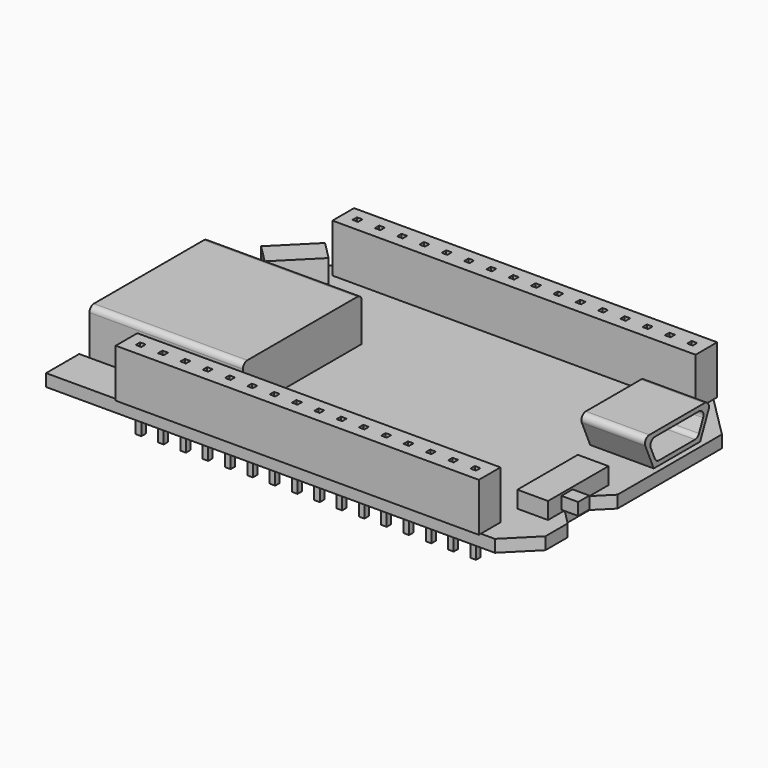
from build123d import *

# Parameters (mm, degrees)
F1_DEPTH  = 1.1
F3_DEPTH  = 1.101
F4_R      = 0.4
F5_DEPTH  = 1.101
F6_W      = 32.55
F6_H      = 2.42
F7_DEPTH  = 4.34
F9_DEPTH  = 2.05
F14_W     = 13.32
F14_H     = 5.65
F15_DEPTH = 9.676
F16_W     = 13.32
F16_H     = 3.93
F17_DEPTH = 4.074
F18_W     = 12.66
F18_H     = 4.99
F18_W_2   = 10.7
F18_H_2   = 2
F19_DEPTH = 8.62
F20_SIZE  = 0.5
F21_R     = 0.5
F11_W     = 2.75
F11_H     = 6.77
F22_DEPTH = 1.5
F26_DEPTH = 5.7
F28_DEPTH = 4
F29_W     = 3.7
F29_H     = 0.8
F30_DEPTH = 2.5
F31_R     = 0.5
F32_W     = 1
F32_H     = 1.45
F33_DEPTH = 0.35
F35_W     = 0.5
F35_H     = 0.5
F36_DEPTH = 3
F37_W     = 0.5
F37_H     = 0.5
F38_DEPTH = 2.7
F39_W     = 1.85
F39_H     = 0.9
F40_DEPTH = 0.7
F41_W     = 1.25
F41_H     = 1.1
F42_DEPTH = 1.5


with BuildPart() as f1:
    # F0 (on Top) → F1 (new body)
    with BuildSketch(Plane.XY):
        Polygon((6.593, 26.37), (0, 19.777), (0, 17.449), (10.426, 17.449), (10.426, 3.714), (0, 3.714), (0, 0), (40.224, 0), (42.743, 2.519), (42.743, 5.019), (41.349, 6.413), (41.349, 9.202), (42.743, 10.596), (42.743, 22.296), (38.669, 26.37), align=None)
    extrude(amount=-F1_DEPTH)

    # F2 (on face) → F3 (cut, through all)
    with BuildSketch(Plane.XY):
        with BuildLine():
            Line((10.426, 16.449), (10.926, 16.449))
            ThreePointArc((10.926, 16.449), (11.426, 16.949), (10.926, 17.449))
            Line((10.926, 17.449), (10.426, 17.449))
            Line((10.426, 17.449), (10.426, 16.449))
        make_face()
        with BuildLine():
            Line((10.426, 3.714), (10.926, 3.714))
            ThreePointArc((10.926, 3.714), (11.426, 4.214), (10.926, 4.714))
            Line((10.926, 4.714), (10.426, 4.714))
            Line((10.426, 4.714), (10.426, 3.714))
        make_face()
    extrude(amount=-F3_DEPTH, mode=Mode.SUBTRACT)

    # F4 (on face) → F5 (cut, through all)
    with BuildSketch(Plane.XY):
        with Locations((7.694, 0.99)):
            Circle(F4_R)
        with Locations((7.694, 25.272)):
            Circle(F4_R)
        with Locations((9.694, 0.99)):
            Circle(F4_R)
        with Locations((9.694, 25.272)):
            Circle(F4_R)
        with Locations((11.694, 0.99)):
            Circle(F4_R)
        with Locations((11.694, 25.272)):
            Circle(F4_R)
        with Locations((13.694, 0.99)):
            Circle(F4_R)
        with Locations((13.694, 25.272)):
            Circle(F4_R)
        with Locations((15.694, 0.99)):
            Circle(F4_R)
        with Locations((15.694, 25.272)):
            Circle(F4_R)
        with Locations((17.694, 0.99)):
            Circle(F4_R)
        with Locations((17.694, 25.272)):
            Circle(F4_R)
        with Locations((19.694, 0.99)):
            Circle(F4_R)
        with Locations((19.694, 25.272)):
            Circle(F4_R)
        with Locations((21.694, 0.99)):
            Circle(F4_R)
        with Locations((21.694, 25.272)):
            Circle(F4_R)
        with Locations((23.694, 0.99)):
            Circle(F4_R)
        with Locations((23.694, 25.272)):
            Circle(F4_R)
        with Locations((25.694, 0.99)):
            Circle(F4_R)
        with Locations((25.694, 25.272)):
            Circle(F4_R)
        with Locations((27.694, 0.99)):
            Circle(F4_R)
        with Locations((27.694, 25.272)):
            Circle(F4_R)
        with Locations((29.694, 0.99)):
            Circle(F4_R)
        with Locations((29.694, 25.272)):
            Circle(F4_R)
        with Locations((31.694, 0.99)):
            Circle(F4_R)
        with Locations((31.694, 25.272)):
            Circle(F4_R)
        with Locations((33.694, 0.99)):
            Circle(F4_R)
        with Locations((33.694, 25.272)):
            Circle(F4_R)
        with Locations((35.694, 0.99)):
            Circle(F4_R)
        with Locations((35.694, 25.272)):
            Circle(F4_R)
        with Locations((37.694, 0.99)):
            Circle(F4_R)
        with Locations((37.694, 25.272)):
            Circle(F4_R)
    extrude(amount=-F5_DEPTH, mode=Mode.SUBTRACT)

    # F25 (on plane+point) → F26 (join, through all)
    with BuildSketch(Plane.YZ.offset(42.243)):
        Polygon((21.734, 2.85), (14.034, 2.85), (15.284, 0), (20.484, 0), align=None)
    extrude(amount=-F26_DEPTH)

    # F27 (on face) → F28 (cut)
    with BuildSketch(Plane.YZ.offset(42.243)):
        Polygon((20.222656384, 0.4), (21.121779191, 2.45), (14.646220809, 2.45), (15.545343616, 0.4), align=None)
    extrude(amount=-F28_DEPTH, mode=Mode.SUBTRACT)

    # F29 (on face) → F30 (join)
    with BuildSketch(Plane.YZ.offset(38.243)):
        with Locations((17.884, 1.8)):
            Rectangle(F29_W, F29_H)
    extrude(amount=F30_DEPTH)

    # F31
    f31_edges = [f1.edges().sort_by_distance(p)[0] for p in [
        (39.393, 14.034, 2.85),
        (39.393, 21.734, 2.85),
        (40.243, 21.121779, 2.45),
        (40.243, 14.646221, 2.45),
        (40.243, 20.222656, 0.4),
        (40.243, 15.545344, 0.4),
    ]]
    fillet(f31_edges, radius=F31_R)


with BuildPart() as f7:
    # F6 (on face) → F7 (new body)
    with BuildSketch(Plane.XY):
        with Locations((22.694, 0.99)):
            Rectangle(F6_W, F6_H)
    extrude(amount=F7_DEPTH)


with BuildPart() as f7b:
    # F6 (on face) → F7, piece 2 (new body)
    with BuildSketch(Plane.XY):
        with Locations((22.694, 25.272)):
            Rectangle(F6_W, F6_H)
    extrude(amount=F7_DEPTH)


with BuildPart() as f9:
    # F8 (on face) → F9 (new body)
    with BuildSketch(Plane.XY):
        Polygon((5.3819805153, 24.5239805153), (2.2, 21.342), (3.8263455967, 19.7156544033), (7.0083261121, 22.8976349186), align=None)
    extrude(amount=F9_DEPTH)

    # F39 (on face) → F40 (join)
    with BuildSketch(Plane(origin=(-9.571, 9.571, 0), x_dir=(-0.7071067812, -0.7071067812, 0), z_dir=(-0.7071067812, 0.7071067812, 0))):
        with Locations((-18.8967078427, 1.025)):
            Rectangle(F39_W, F39_H)
    extrude(amount=F40_DEPTH)


with BuildPart() as f15:
    # F14 (on offset) → F15 (new body, through all)
    with BuildSketch(Plane(origin=(0.75, 0, 0), x_dir=(0, -1, 0), z_dir=(-1, 0, 0))):
        with Locations((-10.5815, 1.105)):
            Rectangle(F14_W, F14_H)
    extrude(amount=-F15_DEPTH)

    # F16 (on face) → F17 (join, through all)
    with BuildSketch(Plane.YZ.offset(10.426)):
        with Locations((10.5815, 1.965)):
            Rectangle(F16_W, F16_H)
    extrude(amount=F17_DEPTH)

    # F18 (on face) → F19 (cut)
    with BuildSketch(Plane(origin=(0.75, 0, 0), x_dir=(0, -1, 0), z_dir=(-1, 0, 0))):
        with Locations((-10.5815, 1.105)):
            Rectangle(F18_W, F18_H)
        with Locations((-10.5815, 2.31)):
            Rectangle(F18_W_2, F18_H_2, mode=Mode.SUBTRACT)
    extrude(amount=-F19_DEPTH, mode=Mode.SUBTRACT)

    # F20
    f20_edges = [f15.edges().sort_by_distance(p)[0] for p in [
        (0.75, 15.9315, 2.31),
        (0.75, 10.5815, 3.31),
        (0.75, 10.5815, 1.31),
        (0.75, 5.2315, 2.31),
    ]]
    chamfer(f20_edges, length=F20_SIZE)

    # F21
    f21_edges = [f15.edges().sort_by_distance(p)[0] for p in [
        (7.625, 17.2415, 3.93),
        (5.06, 16.9115, 3.6),
        (7.625, 3.9215, 3.93),
        (5.06, 4.2515, 3.6),
        (5.06, 4.2515, -1.39),
        (5.06, 16.9115, -1.39),
        (5.588, 17.2415, -1.72),
        (5.588, 3.9215, -1.72),
    ]]
    fillet(f21_edges, radius=F21_R)

    # F32 (on face) → F33 (join)
    with BuildSketch(Plane(origin=(0, 0, -1.72), x_dir=(1, 0, 0), z_dir=(0, 0, -1))):
        with Locations((9.926, -14.0815)):
            Rectangle(F32_W, F32_H)
        with Locations((9.926, -7.0815)):
            Rectangle(F32_W, F32_H)
    extrude(amount=F33_DEPTH)


with BuildPart() as f22:
    # F11 (on face) → F22 (new body)
    with BuildSketch(Plane.XY):
        with Locations((39.974, 7.942)):
            Rectangle(F11_W, F11_H)
    extrude(amount=F22_DEPTH)

    # F41 (on face) → F42 (join)
    with BuildSketch(Plane.YZ.offset(41.349)):
        with Locations((6.682, 0.75)):
            Rectangle(F41_W, F41_H)
    extrude(amount=F42_DEPTH)


with BuildPart() as f36_tool:
    # F35 (on face) → F36 (new body)
    with BuildSketch(Plane.XY.offset(4.34)):
        with Locations((7.694, 0.99)):
            Rectangle(F35_W, F35_H)
        with Locations((7.694, 25.272)):
            Rectangle(F35_W, F35_H)
        with Locations((9.694, 0.99)):
            Rectangle(F35_W, F35_H)
        with Locations((9.694, 25.272)):
            Rectangle(F35_W, F35_H)
        with Locations((11.694, 0.99)):
            Rectangle(F35_W, F35_H)
        with Locations((11.694, 25.272)):
            Rectangle(F35_W, F35_H)
        with Locations((13.694, 0.99)):
            Rectangle(F35_W, F35_H)
        with Locations((13.694, 25.272)):
            Rectangle(F35_W, F35_H)
        with Locations((15.694, 0.99)):
            Rectangle(F35_W, F35_H)
        with Locations((15.694, 25.272)):
            Rectangle(F35_W, F35_H)
        with Locations((17.694, 0.99)):
            Rectangle(F35_W, F35_H)
        with Locations((17.694, 25.272)):
            Rectangle(F35_W, F35_H)
        with Locations((19.694, 0.99)):
            Rectangle(F35_W, F35_H)
        with Locations((19.694, 25.272)):
            Rectangle(F35_W, F35_H)
        with Locations((21.694, 0.99)):
            Rectangle(F35_W, F35_H)
        with Locations((21.694, 25.272)):
            Rectangle(F35_W, F35_H)
        with Locations((23.694, 0.99)):
            Rectangle(F35_W, F35_H)
        with Locations((23.694, 25.272)):
            Rectangle(F35_W, F35_H)
        with Locations((25.694, 0.99)):
            Rectangle(F35_W, F35_H)
        with Locations((25.694, 25.272)):
            Rectangle(F35_W, F35_H)
        with Locations((27.694, 0.99)):
            Rectangle(F35_W, F35_H)
        with Locations((27.694, 25.272)):
            Rectangle(F35_W, F35_H)
        with Locations((29.694, 0.99)):
            Rectangle(F35_W, F35_H)
        with Locations((29.694, 25.272)):
            Rectangle(F35_W, F35_H)
        with Locations((31.694, 0.99)):
            Rectangle(F35_W, F35_H)
        with Locations((31.694, 25.272)):
            Rectangle(F35_W, F35_H)
        with Locations((33.694, 0.99)):
            Rectangle(F35_W, F35_H)
        with Locations((33.694, 25.272)):
            Rectangle(F35_W, F35_H)
        with Locations((35.694, 0.99)):
            Rectangle(F35_W, F35_H)
        with Locations((35.694, 25.272)):
            Rectangle(F35_W, F35_H)
        with Locations((37.694, 0.99)):
            Rectangle(F35_W, F35_H)
        with Locations((37.694, 25.272)):
            Rectangle(F35_W, F35_H)
    extrude(amount=-F36_DEPTH)


with BuildPart() as f7_1:
    add(f7.part)

    # F36: cut by f36_tool
    add(f36_tool.part, mode=Mode.SUBTRACT)

    # F37 (on face) → F38, piece 2 (join, through all)
    with BuildSketch(Plane(origin=(0, 0, 0), x_dir=(1, 0, 0), z_dir=(0, 0, -1))):
        with Locations((37.694, -0.99)):
            Rectangle(F37_W, F37_H)
        with Locations((35.694, -0.99)):
            Rectangle(F37_W, F37_H)
        with Locations((33.694, -0.99)):
            Rectangle(F37_W, F37_H)
        with Locations((31.694, -0.99)):
            Rectangle(F37_W, F37_H)
        with Locations((29.694, -0.99)):
            Rectangle(F37_W, F37_H)
        with Locations((27.694, -0.99)):
            Rectangle(F37_W, F37_H)
        with Locations((25.694, -0.99)):
            Rectangle(F37_W, F37_H)
        with Locations((23.694, -0.99)):
            Rectangle(F37_W, F37_H)
        with Locations((21.694, -0.99)):
            Rectangle(F37_W, F37_H)
        with Locations((19.694, -0.99)):
            Rectangle(F37_W, F37_H)
        with Locations((17.694, -0.99)):
            Rectangle(F37_W, F37_H)
        with Locations((15.694, -0.99)):
            Rectangle(F37_W, F37_H)
        with Locations((13.694, -0.99)):
            Rectangle(F37_W, F37_H)
        with Locations((11.694, -0.99)):
            Rectangle(F37_W, F37_H)
        with Locations((9.694, -0.99)):
            Rectangle(F37_W, F37_H)
        with Locations((7.694, -0.99)):
            Rectangle(F37_W, F37_H)
    extrude(amount=F38_DEPTH)


with BuildPart() as f7b_1:
    add(f7b.part)

    # F36: cut by f36_tool
    add(f36_tool.part, mode=Mode.SUBTRACT)

    # F37 (on face) → F38 (join, through all)
    with BuildSketch(Plane(origin=(0, 0, 0), x_dir=(1, 0, 0), z_dir=(0, 0, -1))):
        with Locations((37.694, -25.272)):
            Rectangle(F37_W, F37_H)
        with Locations((35.694, -25.272)):
            Rectangle(F37_W, F37_H)
        with Locations((33.694, -25.272)):
            Rectangle(F37_W, F37_H)
        with Locations((31.694, -25.272)):
            Rectangle(F37_W, F37_H)
        with Locations((29.694, -25.272)):
            Rectangle(F37_W, F37_H)
        with Locations((27.694, -25.272)):
            Rectangle(F37_W, F37_H)
        with Locations((25.694, -25.272)):
            Rectangle(F37_W, F37_H)
        with Locations((23.694, -25.272)):
            Rectangle(F37_W, F37_H)
        with Locations((21.694, -25.272)):
            Rectangle(F37_W, F37_H)
        with Locations((19.694, -25.272)):
            Rectangle(F37_W, F37_H)
        with Locations((17.694, -25.272)):
            Rectangle(F37_W, F37_H)
        with Locations((15.694, -25.272)):
            Rectangle(F37_W, F37_H)
        with Locations((13.694, -25.272)):
            Rectangle(F37_W, F37_H)
        with Locations((11.694, -25.272)):
            Rectangle(F37_W, F37_H)
        with Locations((9.694, -25.272)):
            Rectangle(F37_W, F37_H)
        with Locations((7.694, -25.272)):
            Rectangle(F37_W, F37_H)
    extrude(amount=F38_DEPTH)


solid = Compound([f1.part, f9.part, f15.part, f22.part, f7_1.part, f7b_1.part])
